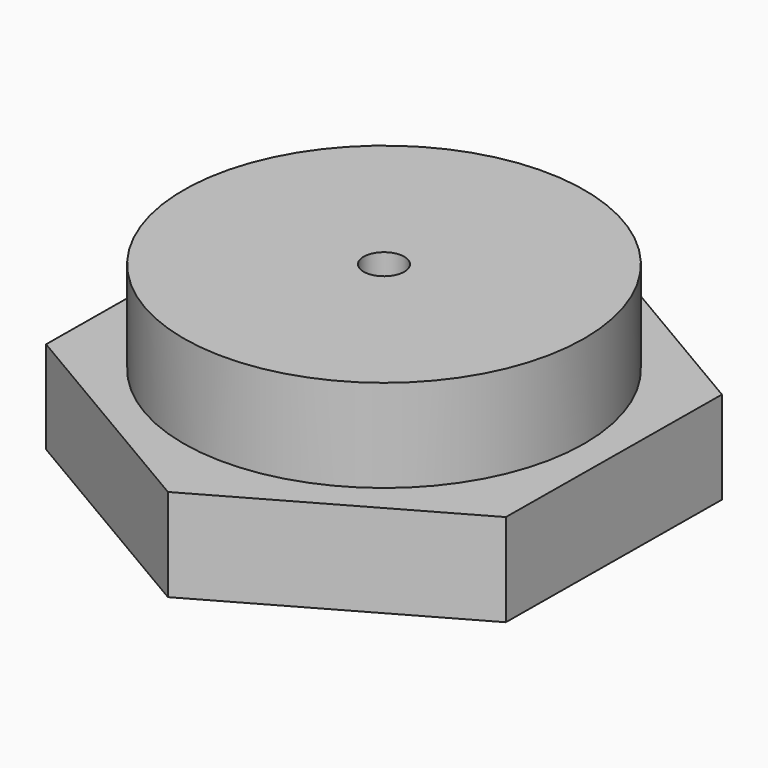
from build123d import *

# Parameters (mm, degrees)
F1_DEPTH = 15
F2_R     = 32.5
F3_DEPTH = 15
F4_R     = 3.3
F5_DEPTH = 30


# Not quite as in the source:
# - a feature names something its author has since deleted; it is built from what else it names


with BuildPart() as f1:
    # F0 (on Top) → F1 (new body)
    with BuildSketch(Plane.XY):
        Polygon((0.369179663, 43.2996963774), (-37.3140472075, 21.9695671555), (-37.6832268705, -21.330129222), (-0.369179663, -43.2996963774), (37.3140472075, -21.9695671555), (37.6832268705, 21.330129222), align=None)
    extrude(amount=F1_DEPTH)

    # F2 (on face) → F3 (join)
    with BuildSketch(Plane.XY.offset(15)):
        Circle(F2_R)
    extrude(amount=F3_DEPTH)


with BuildPart() as f5:
    # F4 (on Top) → F5 (new body)
    with BuildSketch(Plane.XY):
        Circle(F4_R)
    extrude(amount=F5_DEPTH)


with BuildPart() as f1_1:
    add(f1.part)

    # F6: cut F5
    add(f5.part, mode=Mode.SUBTRACT)


solid = f1_1.part
